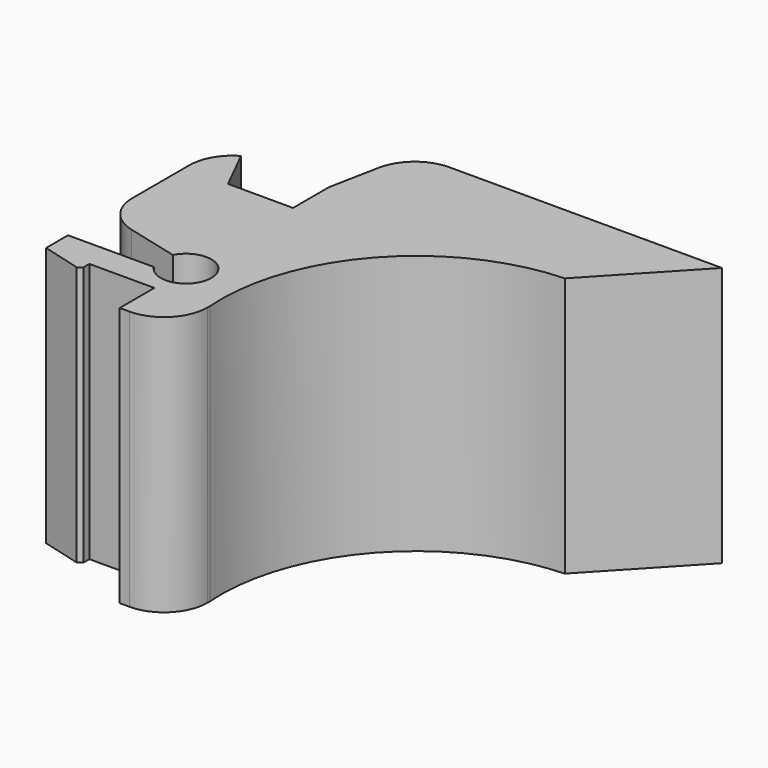
from build123d import *

# Parameters (mm, degrees)
F1_DEPTH    = 12
F2_T1_DEPTH = 22
F2_T3_DEPTH = 20.6602540378
F2_T5_DEPTH = 20.219219555
F2_T7_DEPTH = 19.7630643448
F3_SIZE     = 0.2


# Not quite as in the source:
# - a fillet or chamfer that OpenCascade refuses, or shapes differently, is made with other operations: its cross-section is extruded or revolved along the edge and cut away or added


with BuildPart() as f1:
    # F0 (on Top) → F1 (new body)
    with BuildSketch(Plane.XY):
        with BuildLine():
            Line((0, 17.1366985887), (0, 15.0604258217))
            Line((0, 15.0604258217), (-3, 15.0604258217))
            Line((-3, 15.0604258217), (-4, 17.0604258217))
            Line((-4, 17.0604258217), (-5, 17.0604258217))
            Line((-5, 17.0604258217), (-5, 10.4876235127))
            Line((-5, 10.4876235127), (-1.0879496576, 9.4864424318))
            ThreePointArc((-1.0879496576, 9.4864424318), (1.1165361393, 8.9993738808), (-1.0382550692, 8.3256764337))
            Line((-1.0382550692, 8.3256764337), (-5, 8.3256764337))
            Line((-5, 8.3256764337), (-5, 7.6356520876))
            Line((-5, 7.6356520876), (-5, 7.0604258217))
            Line((-5, 7.0604258217), (-3, 6.5184039995))
            Line((-3, 6.5184039995), (-3, 7.0604258217))
            Line((-3, 7.0604258217), (0, 7.0604258217))
            Line((0, 7.0604258217), (0, 5.0604258217))
            Line((0, 5.0604258217), (2.4494461788, 5.0604258217))
            Line((2.4494461788, 5.0604258217), (2.4494461788, 7.2136978708))
            ThreePointArc((2.4494461788, 7.2136978708), (4.7188246076, 13.8799594264), (11.0867818181, 16.8863264277))
            Line((11.0867818181, 16.8863264277), (15, 21.0604258217))
            Line((15, 21.0604258217), (2.1266145632, 21.0604258217))
            Line((2.1266145632, 21.0604258217), (0.7744232425, 21.0604258217))
            Line((0.7744232425, 21.0604258217), (0, 17.1366985887))
        make_face()
    extrude(amount=F1_DEPTH)

    # F2: fillet of radius 2 on 4 edges, made by hand

    # F2_s2 → F2_t1 (cut)
    with BuildSketch(Plane.XY.offset(-5)):
        with BuildLine():
            ThreePointArc((2.4494461788, 7.0604258217), (1.8636597412, 5.6462122593), (0.4494461788, 5.0604258217))
            Line((0.4494461788, 5.0604258217), (2.4494461788, 5.0604258217))
            Line((2.4494461788, 5.0604258217), (2.4494461788, 7.0604258217))
        make_face()
    extrude(amount=F2_T1_DEPTH, mode=Mode.SUBTRACT)

    # F2_s4 → F2_t3 (cut)
    with BuildSketch(Plane.XY.offset(-4.3301270189)):
        with BuildLine():
            ThreePointArc((-5, 15.3283750141), (-4.7320508076, 16.3283750141), (-4, 17.0604258217))
            Line((-4, 17.0604258217), (-5, 17.0604258217))
            Line((-5, 17.0604258217), (-5, 15.3283750141))
        make_face()
    extrude(amount=F2_T3_DEPTH, mode=Mode.SUBTRACT)

    # F2_s6 → F2_t5 (cut)
    with BuildSketch(Plane.XY.offset(-4.1096097775)):
        with BuildLine():
            ThreePointArc((2.4182671536, 21.0604258217), (1.1483331779, 20.6055043625), (0.4561194194, 19.4476935191))
            Line((0.4561194194, 19.4476935191), (0.7744232425, 21.0604258217))
            Line((0.7744232425, 21.0604258217), (2.4182671536, 21.0604258217))
        make_face()
    extrude(amount=F2_T5_DEPTH, mode=Mode.SUBTRACT)

    # F2_s8 → F2_t7 (cut)
    with BuildSketch(Plane.XY.offset(-3.8815321724)):
        with BuildLine():
            ThreePointArc((-3.4958636049, 10.1026814056), (-4.5798302456, 10.8138039967), (-5, 12.0402363817))
            Line((-5, 12.0402363817), (-5, 10.4876235127))
            Line((-5, 10.4876235127), (-3.4958636049, 10.1026814056))
        make_face()
    extrude(amount=F2_T7_DEPTH, mode=Mode.SUBTRACT)

    # F3
    f3_edges = [f1.edges().sort_by_distance(p)[0] for p in [
        (-3, 6.518404, 6),
    ]]
    chamfer(f3_edges, length=F3_SIZE)


solid = f1.part
